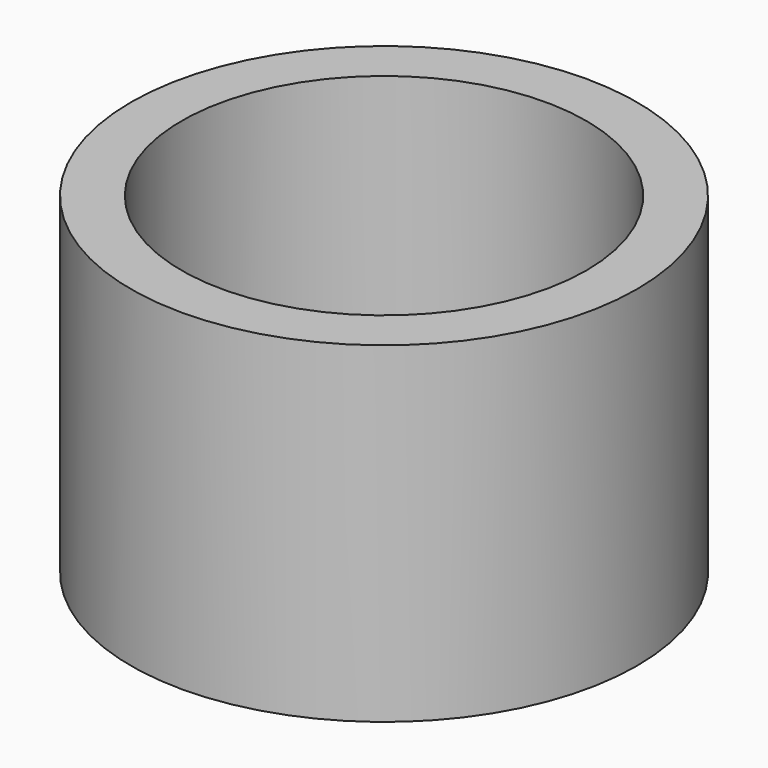
from build123d import *

# Parameters (mm, degrees)
F0_R         = 14.5
F1_DEPTH     = 19
F2_R         = 11.6
F3_DEPTH     = 15
F4_TEXT_SIZE = 13.8888888889
F5_DEPTH     = 1


# Not quite as in the source:
# - Text() gives the source's letters only with a copy of the font that has no kerning and outlines rounded to 1/6400 em; it was checked with that copy


with BuildPart() as f1:
    # F0 (on Top) → F1 (new body)
    with BuildSketch(Plane.XY):
        Circle(F0_R)
    extrude(amount=F1_DEPTH)

    # F2 (on face) → F3 (cut)
    with BuildSketch(Plane.XY.offset(19)):
        Circle(F2_R)
    extrude(amount=-F3_DEPTH, mode=Mode.SUBTRACT)

    # F4 (on face) → F5 (cut)
    with BuildSketch(Plane(origin=(0, 0, 0), x_dir=(1, 0, 0), z_dir=(0, 0, -1))):
        with Locations((-8.951314175, -4.9803546404)):
            Text('PP', F4_TEXT_SIZE, font='Open Sans', font_style=FontStyle.BOLD, text_align=(TextAlign.LEFT, TextAlign.BOTTOM))
    extrude(amount=-F5_DEPTH, mode=Mode.SUBTRACT)


solid = f1.part
